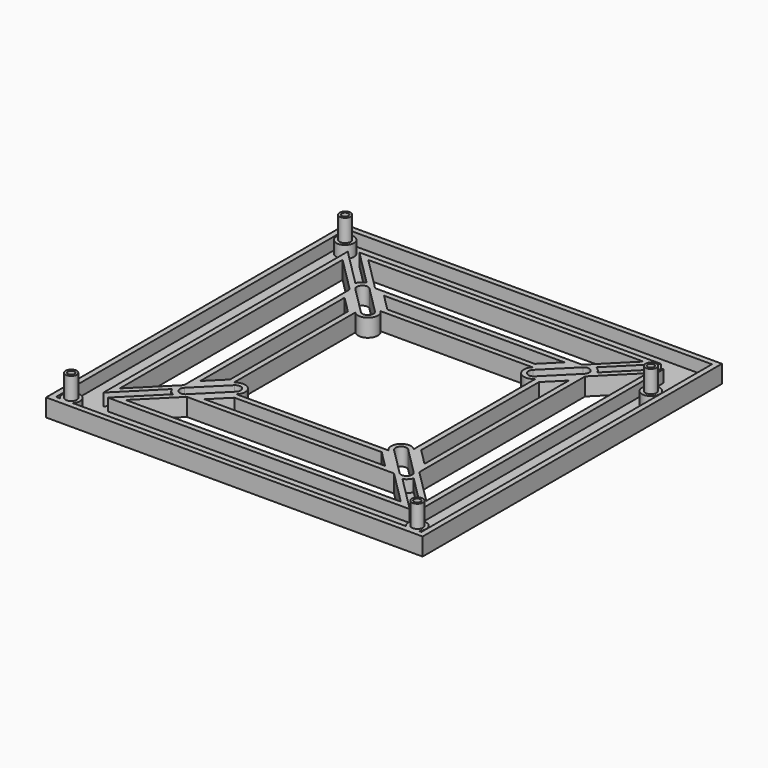
from build123d import *

# Parameters (mm, degrees)
F0_W        = 170.1745619284
F0_H        = 169.0850543895
F0_R        = 2.5
F0_R_2      = 1.5
F1_DEPTH    = 8
F2_T        = 2.5
F2_T3_DEPTH = 13
F3_R        = 2.5
F3_R_2      = 1.5
F4_DEPTH    = 10


# Not quite as in the source:
# - a shell that OpenCascade refuses in one call is made with other operations: the cavity is built on its own and cut out


with BuildPart() as f1:
    # F0 (on Top) → F1 (new body)
    with BuildSketch(Plane.XY):
        with Locations((57.8983475621, -0.8945845068)):
            Rectangle(F0_W, F0_H)
        with Locations((-20.0254507363, -80.1839753985)):
            Circle(F0_R, mode=Mode.SUBTRACT)
        with Locations((136.3779287785, -80.1476985216)):
            Circle(F0_R, mode=Mode.SUBTRACT)
        with Locations((-20.0218968093, 74.5575577021)):
            Circle(F0_R, mode=Mode.SUBTRACT)
        Polygon((-11.1889293083, 67.6479385942), (-4.0385814859, 67.6479385942), (120.3185426547, 67.6479385942), (126.9856244326, 67.6479385942), (126.9856244326, 61.5870983108), (126.9856244326, -63.3762673243), (126.9856244326, -69.4371076077), (120.3185426547, -69.4371076077), (-4.0385814859, -69.4371076077), (-11.1889293083, -69.4371076077), (-11.1889293083, -63.8595333687), (-11.1889293083, 62.0703643552), align=None, mode=Mode.SUBTRACT)
        with Locations((136.3756339997, 51.792871207)):
            Circle(F0_R, mode=Mode.SUBTRACT)
        with BuildLine():
            Line((23.8219610997, 39.7873960086), (11.3219610997, 52.2873960086))
            ThreePointArc((11.3219610997, 52.2873960086), (4.958000069, 52.2873960086), (4.958000069, 45.9234349779))
            Line((4.958000069, 45.9234349779), (17.458000069, 33.4234349779))
            ThreePointArc((17.458000069, 33.4234349779), (23.8219610997, 33.4234349779), (23.8219610997, 39.7873960086))
        make_face()
        with BuildLine():
            ThreePointArc((22.4077475373, 38.3731824462), (22.4077475373, 34.8376485403), (18.8722136314, 34.8376485403))
            Line((18.8722136314, 34.8376485403), (6.3722136314, 47.3376485403))
            ThreePointArc((6.3722136314, 47.3376485403), (6.3722136314, 50.8731824462), (9.9077475373, 50.8731824462))
            Line((9.9077475373, 50.8731824462), (22.4077475373, 38.3731824462))
        make_face(mode=Mode.SUBTRACT)
        with BuildLine():
            ThreePointArc((111.3219610997, 45.9234349779), (111.3219610997, 52.2873960086), (104.958000069, 52.2873960086))
            Line((104.958000069, 52.2873960086), (92.458000069, 39.7873960086))
            ThreePointArc((92.458000069, 39.7873960086), (92.458000069, 33.4234349779), (98.8219610997, 33.4234349779))
            Line((98.8219610997, 33.4234349779), (111.3219610997, 45.9234349779))
        make_face()
        with BuildLine():
            Line((109.9077475373, 47.3376485403), (97.4077475373, 34.8376485403))
            ThreePointArc((97.4077475373, 34.8376485403), (93.8722136314, 34.8376485403), (93.8722136314, 38.3731824462))
            Line((93.8722136314, 38.3731824462), (106.3722136314, 50.8731824462))
            ThreePointArc((106.3722136314, 50.8731824462), (109.9077475373, 50.8731824462), (109.9077475373, 47.3376485403))
        make_face(mode=Mode.SUBTRACT)
        with BuildLine():
            ThreePointArc((104.958000069, -54.0765650221), (111.3219610997, -54.0765650221), (111.3219610997, -47.7126039914))
            Line((111.3219610997, -47.7126039914), (98.8219610997, -35.2126039914))
            ThreePointArc((98.8219610997, -35.2126039914), (92.458000069, -35.2126039914), (92.458000069, -41.5765650221))
            Line((92.458000069, -41.5765650221), (104.958000069, -54.0765650221))
        make_face()
        with BuildLine():
            ThreePointArc((93.8722136314, -40.1623514597), (93.8722136314, -36.6268175538), (97.4077475373, -36.6268175538))
            Line((97.4077475373, -36.6268175538), (109.9077475373, -49.1268175538))
            ThreePointArc((109.9077475373, -49.1268175538), (109.9077475373, -52.6623514597), (106.3722136314, -52.6623514597))
            Line((106.3722136314, -52.6623514597), (93.8722136314, -40.1623514597))
        make_face(mode=Mode.SUBTRACT)
        with BuildLine():
            Line((17.458000069, -35.2126039914), (4.958000069, -47.7126039914))
            ThreePointArc((4.958000069, -47.7126039914), (4.958000069, -54.0765650221), (11.3219610997, -54.0765650221))
            Line((11.3219610997, -54.0765650221), (23.8219610997, -41.5765650221))
            ThreePointArc((23.8219610997, -41.5765650221), (23.8219610997, -35.2126039914), (17.458000069, -35.2126039914))
        make_face()
        with BuildLine():
            Line((6.3722136314, -49.1268175538), (18.8722136314, -36.6268175538))
            ThreePointArc((18.8722136314, -36.6268175538), (22.4077475373, -36.6268175538), (22.4077475373, -40.1623514597))
            Line((22.4077475373, -40.1623514597), (9.9077475373, -52.6623514597))
            ThreePointArc((9.9077475373, -52.6623514597), (6.3722136314, -52.6623514597), (6.3722136314, -49.1268175538))
        make_face(mode=Mode.SUBTRACT)
        with Locations((-20.0218968093, 74.5575577021)):
            Circle(F0_R)
        with Locations((-20.0218968093, 74.5575577021)):
            Circle(F0_R_2, mode=Mode.SUBTRACT)
        with Locations((136.3756339997, 51.792871207)):
            Circle(F0_R)
        with Locations((136.3756339997, 51.792871207)):
            Circle(F0_R_2, mode=Mode.SUBTRACT)
        with Locations((136.3779287785, -80.1476985216)):
            Circle(F0_R)
        with Locations((136.3779287785, -80.1476985216)):
            Circle(F0_R_2, mode=Mode.SUBTRACT)
        with Locations((-20.0254507363, -80.1839753985)):
            Circle(F0_R)
        with Locations((-20.0254507363, -80.1839753985)):
            Circle(F0_R_2, mode=Mode.SUBTRACT)
        with BuildLine():
            Line((126.9856244326, -63.3762673243), (111.3219610997, -47.7126039914))
            ThreePointArc((111.3219610997, -47.7126039914), (111.3219610997, -54.0765650221), (104.958000069, -54.0765650221))
            Line((104.958000069, -54.0765650221), (120.3185426547, -69.4371076077))
            Line((120.3185426547, -69.4371076077), (126.9856244326, -69.4371076077))
            Line((126.9856244326, -69.4371076077), (126.9856244326, -63.3762673243))
        make_face()
        with BuildLine():
            ThreePointArc((11.3219610997, -54.0765650221), (4.958000069, -54.0765650221), (4.958000069, -47.7126039914))
            Line((4.958000069, -47.7126039914), (-11.1889293083, -63.8595333687))
            Line((-11.1889293083, -63.8595333687), (-11.1889293083, -69.4371076077))
            Line((-11.1889293083, -69.4371076077), (-4.0385814859, -69.4371076077))
            Line((-4.0385814859, -69.4371076077), (11.3219610997, -54.0765650221))
        make_face()
        Polygon((23.8219610997, -41.5765650221), (11.3219610997, -54.0765650221), (104.958000069, -54.0765650221), (92.458000069, -41.5765650221), align=None)
        Polygon((24.857495267, -44.0765656531), (91.4224659017, -44.0765656531), (98.9224646398, -51.5765643911), (17.357496529, -51.5765643911), align=None, mode=Mode.SUBTRACT)
        Polygon((111.3219610997, -47.7126039914), (111.3219610997, 45.9234349779), (98.8219610997, 33.4234349779), (98.8219610997, -35.2126039914), align=None)
        Polygon((101.3219610997, -34.1770700855), (101.3219610997, 32.387901072), (108.8219610997, 39.887901072), (108.8219610997, -41.6770700855), align=None, mode=Mode.SUBTRACT)
        Polygon((17.458000069, 33.4234349779), (4.958000069, 45.9234349779), (4.958000069, -47.7126039914), (17.458000069, -35.2126039914), align=None)
        Polygon((14.958000069, 32.387901072), (14.958000069, -34.1770700855), (7.458000069, -41.6770700855), (7.458000069, 39.887901072), align=None, mode=Mode.SUBTRACT)
        Polygon((104.958000069, 52.2873960086), (11.3219610997, 52.2873960086), (23.8219610997, 39.7873960086), (92.458000069, 39.7873960086), align=None)
        Polygon((91.4224661631, 42.2873960086), (24.8574950057, 42.2873960086), (17.3574950057, 49.7873960086), (98.9224661631, 49.7873960086), align=None, mode=Mode.SUBTRACT)
        with BuildLine():
            Line((120.3185426547, 67.6479385942), (104.958000069, 52.2873960086))
            ThreePointArc((104.958000069, 52.2873960086), (111.3219610997, 52.2873960086), (111.3219610997, 45.9234349779))
            Line((111.3219610997, 45.9234349779), (126.9856244326, 61.5870983108))
            Line((126.9856244326, 61.5870983108), (126.9856244326, 67.6479385942))
            Line((126.9856244326, 67.6479385942), (120.3185426547, 67.6479385942))
        make_face()
        with BuildLine():
            ThreePointArc((4.958000069, 45.9234349779), (4.958000069, 52.2873960086), (11.3219610997, 52.2873960086))
            Line((11.3219610997, 52.2873960086), (-4.0385814859, 67.6479385942))
            Line((-4.0385814859, 67.6479385942), (-11.1889293083, 67.6479385942))
            Line((-11.1889293083, 67.6479385942), (-11.1889293083, 62.0703643552))
            Line((-11.1889293083, 62.0703643552), (4.958000069, 45.9234349779))
        make_face()
    extrude(amount=F1_DEPTH)

    # F2: shell of thickness 2.5, made by hand


with BuildPart() as f2_core1:
    # F2_t2: copy of F1
    add(f1.part)

    # the walls: a layer under each face that stays
    f2_faces = [f2_core1.faces().sort_by_distance(p)[0] for p in [
        (57.8983475621, 83.647942688, 4),
        (-27.1889334021, -0.8945845068, 4),
        (57.8983475621, -85.4371117015, 4),
        (142.9856285263, -0.8945845068, 4),
        (58.1399805844, 67.6479385942, 4),
        (112.6382713619, 59.9676673014, 4),
        (58.1399805844, 52.2873960086, 4),
        (3.6416898069, 59.9676673014, 4),
        (4.958000069, -0.8945845068, 4),
        (-3.1154646196, -55.7860686801, 4),
        (-11.1889293083, -0.8945845067, 4),
        (-3.1154646196, 53.9968996666, 4),
        (126.9856244326, -0.8945845068, 4),
        (119.1537927661, -55.5444356578, 4),
        (111.3219610997, -0.8945845068, 4),
        (119.1537927661, 53.7552666443, 4),
        (92.458000069, 33.4234349779, 4),
        (98.8219610997, -0.8945845068, 4),
        (92.458000069, -35.2126039914, 4),
        (58.1399805844, -41.5765650221, 4),
        (23.8219610997, -35.2126039914, 4),
        (17.458000069, -0.8945845068, 4),
        (23.8219610997, 33.4234349779, 4),
        (58.1399805844, 39.7873960086, 4),
        (112.6382713619, -61.7568363149, 4),
        (58.1399805844, -69.4371076077, 4),
        (3.6416898069, -61.7568363149, 4),
        (58.1399805844, -54.0765650221, 4),
        (-21.5218968093, 74.5575577021, 4),
        (134.8756339997, 51.792871207, 4),
        (134.8779287785, -80.1476985216, 4),
        (-21.5254507363, -80.1839753985, 4),
        (103.6577475373, -42.8768175538, 4),
        (109.9077475373, -52.6623514597, 4),
        (100.1222136314, -46.4123514597, 4),
        (93.8722136314, -36.6268175538, 4),
        (16.1577475373, -46.4123514597, 4),
        (6.3722136314, -52.6623514597, 4),
        (12.6222136314, -42.8768175538, 4),
        (22.4077475373, -36.6268175538, 4),
        (58.1399805844, -51.5765643911, 4),
        (21.107495898, -47.8265650221, 4),
        (58.1399805844, -44.0765656531, 4),
        (95.1724652707, -47.8265650221, 4),
        (108.8219610997, -0.8945845068, 4),
        (105.0719610997, -37.9270700855, 4),
        (101.3219610997, -0.8945845068, 4),
        (105.0719610997, 36.137901072, 4),
        (109.9077475373, 50.8731824462, 4),
        (103.6577475373, 41.0876485403, 4),
        (93.8722136314, 34.8376485403, 4),
        (100.1222136314, 44.6231824462, 4),
        (7.458000069, -0.8945845068, 4),
        (11.208000069, 36.137901072, 4),
        (14.958000069, -0.8945845068, 4),
        (11.208000069, -37.9270700855, 4),
        (6.3722136314, 50.8731824462, 4),
        (16.1577475373, 44.6231824462, 4),
        (22.4077475373, 34.8376485403, 4),
        (12.6222136314, 41.0876485403, 4),
        (58.1399805844, 42.2873960086, 4),
        (21.1074950057, 46.0373960086, 4),
        (58.1399805844, 49.7873960086, 4),
        (95.1724661631, 46.0373960086, 4),
        (1.173493586, -57.2562693032, 0),
    ]]
    thicken(f2_faces, amount=-F2_T, mode=Mode.SUBTRACT)

    # F2_s4 → F2_t3 (cut)
    with BuildSketch(Plane.XY.offset(-2.5)):
        Polygon((-4.0209038164, 67.6406162638), (-4.0385814859, 70.1479385942), (-10.0741153918, 70.1479385942), (-5.8063484389, 65.8801716413), align=None)
        Polygon((120.3008649852, 67.6406162638), (120.3185426547, 70.1479385942), (126.3540765606, 70.1479385942), (122.0863096076, 65.8801716413), align=None)
        Polygon((104.9403223995, 52.3300736781), (106.725767022, 50.5196290556), (105.993533975, 49.7873960086), (104.958000069, 49.7873960086), align=None)
        Polygon((11.3396387693, 52.3300736781), (11.3219610997, 49.7873960086), (10.2864271938, 49.7873960086), (9.5541941468, 50.5196290556), align=None)
        Polygon((4.9153223995, 45.9057573084), (7.458000069, 45.9234349779), (7.458000069, 46.9589688838), (6.725767022, 47.6912019309), align=None)
        Polygon((4.9153223995, -47.6949263219), (7.458000069, -47.7126039914), (7.458000069, -48.7481378973), (6.725767022, -49.4803709444), align=None)
        Polygon((-11.1816069778, -63.8418556992), (-9.4211623553, -65.6273003217), (-13.6889293083, -69.8950672747), (-13.6889293083, -63.8595333687), align=None)
        Polygon((-11.1816069778, 62.0526866857), (-13.6889293083, 62.0703643552), (-13.6889293083, 68.1058982612), (-9.4211623553, 63.8381313082), align=None)
        Polygon((126.9783021021, 61.5694206412), (129.4856244326, 61.5870983108), (129.4856244326, 67.6226322167), (125.2178574796, 63.3548652637), align=None)
        Polygon((126.9783021021, -63.3585896547), (129.4856244326, -63.3762673243), (129.4856244326, -69.4118012302), (125.2178574796, -65.1440342772), align=None)
        Polygon((111.3646387693, -47.6949263219), (109.5541941468, -49.4803709444), (108.8219610997, -48.7481378973), (108.8219610997, -47.7126039914), align=None)
        Polygon((111.3646387693, 45.9057573084), (108.8219610997, 45.9234349779), (108.8219610997, 46.9589688838), (109.5541941468, 47.6912019309), align=None)
        Polygon((92.4403223995, 39.7800736781), (94.225767022, 38.0196290556), (98.493533975, 42.2873960086), (92.458000069, 42.2873960086), align=None)
        Polygon((98.8146387693, 33.4057573084), (97.0541941468, 35.1912019309), (101.3219610997, 39.4589688838), (101.3219610997, 33.4234349779), align=None)
        Polygon((98.8146387693, -35.1949263219), (101.3219610997, -35.2126039914), (101.3219610997, -41.2481378973), (97.0541941468, -36.9803709444), align=None)
        Polygon((92.4403223995, -41.5692426916), (94.225767022, -39.8087980691), (98.493533975, -44.0765650221), (92.458000069, -44.0765650221), align=None)
        Polygon((23.8396387693, -41.5692426916), (23.8219610997, -44.0765650221), (17.7864271938, -44.0765650221), (22.0541941468, -39.8087980691), align=None)
        Polygon((17.4653223995, -35.1949263219), (19.225767022, -36.9803709444), (14.958000069, -41.2481378973), (14.958000069, -35.2126039914), align=None)
        Polygon((17.4653223995, 33.4057573084), (14.958000069, 33.4234349779), (14.958000069, 39.4589688838), (19.225767022, 35.1912019309), align=None)
        Polygon((23.8396387693, 39.7800736781), (22.0541941468, 38.0196290556), (17.7864271938, 42.2873960086), (23.8219610997, 42.2873960086), align=None)
        Polygon((104.9403223995, -54.1192426916), (106.725767022, -52.3087980691), (105.993533975, -51.5765650221), (104.958000069, -51.5765650221), align=None)
        Polygon((120.3008649852, -69.4297852773), (122.0863096076, -67.6693406548), (126.3540765606, -71.9371076077), (120.3185426547, -71.9371076077), align=None)
        Polygon((-4.0209038164, -69.4297852773), (-4.0385814859, -71.9371076077), (-10.0741153918, -71.9371076077), (-5.8063484389, -67.6693406548), align=None)
        Polygon((11.3396387693, -54.1192426916), (9.5541941468, -52.3087980691), (10.2864271938, -51.5765650221), (11.3219610997, -51.5765650221), align=None)
        Polygon((98.9047869702, -51.5692420606), (98.9224646398, -54.0765643911), (104.9579985457, -54.0765643911), (100.6902315927, -49.8087974381), align=None)
        Polygon((17.3751741985, -51.5692420606), (17.357496529, -54.0765643911), (11.3219626231, -54.0765643911), (15.589729576, -49.8087974381), align=None)
        Polygon((24.8751729366, -44.1192433226), (23.0897283141, -42.3087987001), (23.8219613611, -41.5765656531), (24.857495267, -41.5765656531), align=None)
        Polygon((91.4047882322, -44.1192433226), (91.4224659017, -41.5765656531), (92.4579998077, -41.5765656531), (93.1902328547, -42.3087987001), align=None)
        Polygon((108.8146387693, 39.8702234024), (111.3219610997, 39.887901072), (111.3219610997, 45.9234349779), (107.0541941468, 41.6556680249), align=None)
        Polygon((108.8146387693, -41.6593924159), (111.3219610997, -41.6770700855), (111.3219610997, -47.7126039914), (107.0541941468, -43.4448370384), align=None)
        Polygon((101.3646387693, -34.1593924159), (99.5541941468, -35.9448370384), (98.8219610997, -35.2126039914), (98.8219610997, -34.1770700855), align=None)
        Polygon((101.3646387693, 32.3702234024), (98.8219610997, 32.387901072), (98.8219610997, 33.4234349779), (99.5541941468, 34.1556680249), align=None)
        Polygon((7.4653223995, -41.6593924159), (4.958000069, -41.6770700855), (4.958000069, -47.7126039914), (9.225767022, -43.4448370384), align=None)
        Polygon((7.4653223995, 39.8702234024), (4.958000069, 39.887901072), (4.958000069, 45.9234349779), (9.225767022, 41.6556680249), align=None)
        Polygon((14.9153223995, 32.3702234024), (16.725767022, 34.1556680249), (17.458000069, 33.4234349779), (17.458000069, 32.387901072), align=None)
        Polygon((14.9153223995, -34.1593924159), (17.458000069, -34.1770700855), (17.458000069, -35.2126039914), (16.725767022, -35.9448370384), align=None)
        Polygon((91.4047884936, 42.3300736781), (91.4224661631, 39.7873960086), (92.458000069, 39.7873960086), (93.1902331161, 40.5196290556), align=None)
        Polygon((24.8751726752, 42.3300736781), (24.8574950057, 39.7873960086), (23.8219610997, 39.7873960086), (23.0897280527, 40.5196290556), align=None)
        Polygon((17.3751726752, 49.7800736781), (15.5897280527, 48.0196290556), (11.3219610997, 52.2873960086), (17.3574950057, 52.2873960086), align=None)
        Polygon((98.9047884936, 49.7800736781), (98.9224661631, 52.2873960086), (104.958000069, 52.2873960086), (100.6902331161, 48.0196290556), align=None)
    extrude(amount=F2_T3_DEPTH, mode=Mode.SUBTRACT)


with BuildPart() as f1_1:
    add(f1.part)

    # what is left inside the walls is the cavity
    f2_cavity = [f2_core1.part.solids().sort_by_distance(p)[0] for p in [
        (-14.365523, 62.91627, 2.525),
    ]]
    add(f2_cavity, mode=Mode.SUBTRACT)

    # F3 (on face) → F4 (join)
    with BuildSketch(Plane.XY.offset(8)):
        with Locations((136.3756339997, 51.792871207)):
            Circle(F3_R)
        with Locations((136.3756339997, 51.792871207)):
            Circle(F3_R_2, mode=Mode.SUBTRACT)
        with Locations((-20.0218968093, 74.5575577021)):
            Circle(F3_R)
        with Locations((-20.0218968093, 74.5575577021)):
            Circle(F3_R_2, mode=Mode.SUBTRACT)
        with Locations((-20.0254507363, -80.1839753985)):
            Circle(F3_R)
        with Locations((-20.0254507363, -80.1839753985)):
            Circle(F3_R_2, mode=Mode.SUBTRACT)
        with Locations((136.3779287785, -80.1476985216)):
            Circle(F3_R)
        with Locations((136.3779287785, -80.1476985216)):
            Circle(F3_R_2, mode=Mode.SUBTRACT)
    extrude(amount=F4_DEPTH)


solid = f1_1.part
